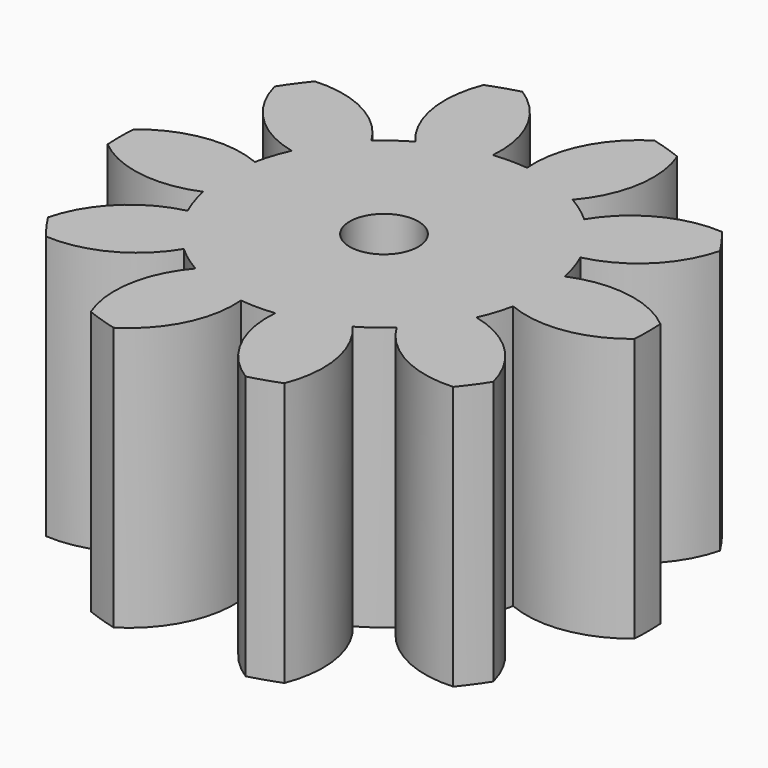
from build123d import *

# Parameters (mm, degrees)
F0_R            = 5
F0_R_2          = 0.65
F1_DEPTH        = 5
F3_DEPTH        = 25
F3_COPIES_COUNT = 10


# Not quite as in the source:
# - a feature of the source that left no trace in its solid (it failed there, or was rolled back) is left out
# - a pattern or mirror of a feature is missing from the dataset's text; its kind, count and spacing are read off the source's solid


with BuildPart() as f1:
    # F0 (on Top) → F1 (new body)
    with BuildSketch(Plane.XY):
        Circle(F0_R)
        Circle(F0_R_2, mode=Mode.SUBTRACT)
    extrude(amount=F1_DEPTH)

    # F2 (on face) → F3 (cut)
    with BuildSketch(Plane.XY.offset(5)):
        with BuildLine():
            ThreePointArc((-0.325, 2.9823438769), (0, 3), (0.325, 2.9823438769))
            ThreePointArc((0.325, 2.9823438769), (0.5273788104, 4.0412254466), (1.25, 4.8412291828))
            ThreePointArc((1.25, 4.8412291828), (0, 5), (-1.25, 4.8412291828))
            ThreePointArc((-1.25, 4.8412291828), (-0.5273788104, 4.0412254466), (-0.325, 2.9823438769))
        make_face()
    f3 = extrude(amount=-F3_DEPTH, mode=Mode.SUBTRACT)

    # F3_copies: F3 ×10 about axis
    f3_copies_axis = Axis((0, 0, 0), (0, 0, 1))
    for i in range(1, F3_COPIES_COUNT):
        add(f3.rotate(f3_copies_axis, i * 360 / F3_COPIES_COUNT), mode=Mode.SUBTRACT)


solid = f1.part
